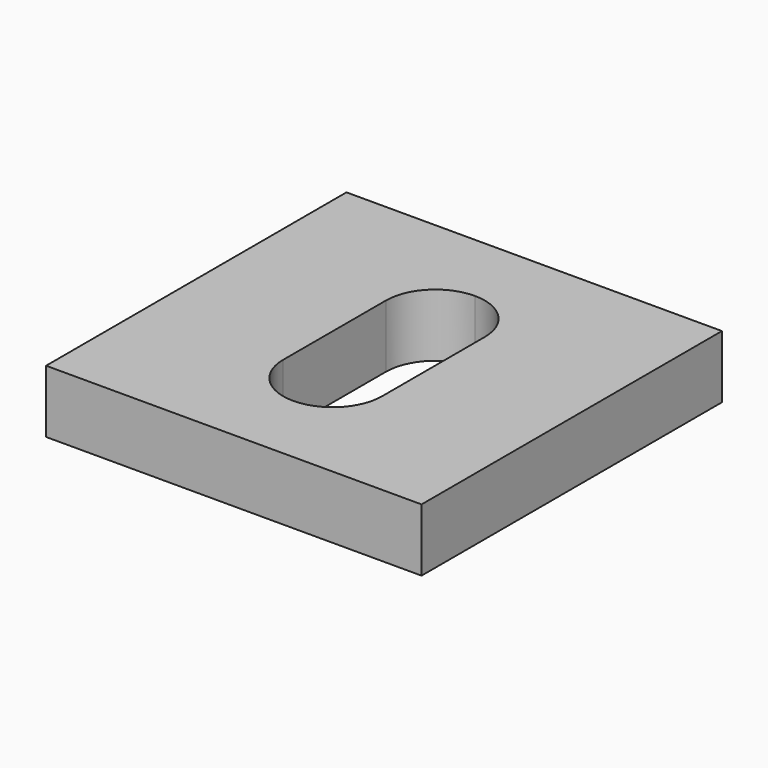
from build123d import *

# Parameters (mm, degrees)
F0_W     = 19
F0_H     = 19
F0_W_2   = 5
F0_H_2   = 11.5
F1_DEPTH = 3.175
F2_R     = 2.49999


# Not quite as in the source:
# - a fillet or chamfer is up to 0.001 mm smaller than in the source, because OpenCascade refuses the exact size


with BuildPart() as f1:
    # F0 (on Top) → F1 (new body)
    with BuildSketch(Plane.XY):
        Rectangle(F0_W, F0_H)
        Rectangle(F0_W_2, F0_H_2, mode=Mode.SUBTRACT)
    extrude(amount=F1_DEPTH)

    # F2 (radius 2.5 in the source; OpenCascade refuses exactly that, so slightly less here)
    f2_edges = [f1.edges().sort_by_distance(p)[0] for p in [
        (-2.5, 5.75, 1.5875),
        (-2.5, -5.75, 1.5875),
        (2.5, 5.75, 1.5875),
        (2.5, -5.75, 1.5875),
    ]]
    fillet(f2_edges, radius=F2_R)


solid = f1.part
